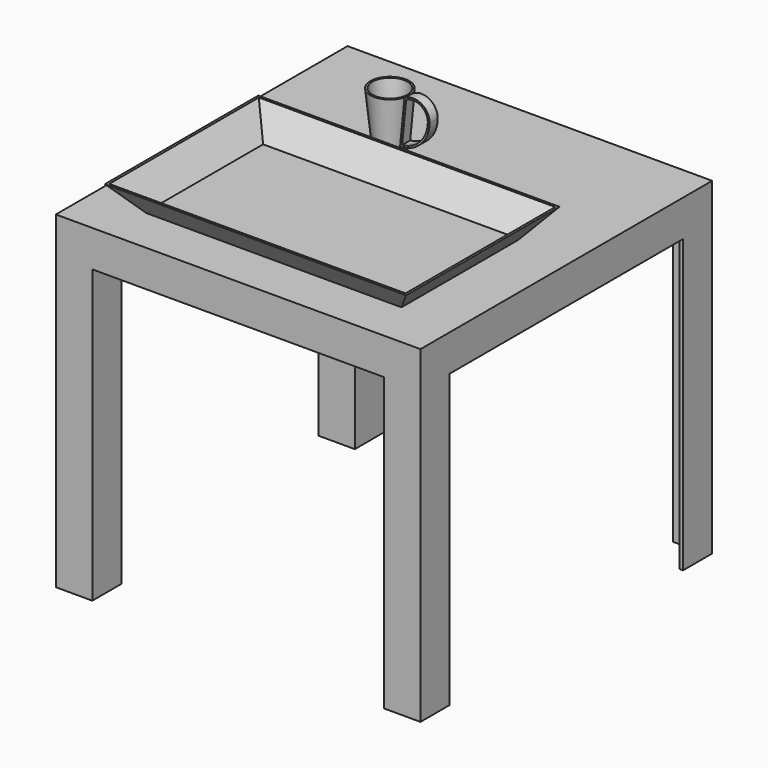
from build123d import *

# Parameters (mm, degrees)
F0_W         = 508
F0_H         = 457.2
F1_DEPTH     = 508
F3_DEPTH     = 406.4
F4_T         = 5.08
F4_T3_DEPTH  = 60.96
F4_T5_DEPTH  = 60.96
F4_T7_DEPTH  = 60.96
F4_T9_DEPTH  = 60.96
F5_R         = 19.05
F6_DEPTH     = 76.2
F6_TAPER     = -6
F7_T         = 2.54
F7_T3_DEPTH  = 55.88
F7_T5_DEPTH  = 55.88
F7_T7_DEPTH  = 55.88
F7_T9_DEPTH  = 10.16
F7_T11_DEPTH = 10.16
F7_T13_DEPTH = 55.88
F7_T15_DEPTH = 10.16
F7_T17_DEPTH = 457.2
F7_T19_DEPTH = 416.56
F7_T21_DEPTH = 411.48
F7_T23_DEPTH = 45.72
F7_T25_DEPTH = 452.12
F7_T27_DEPTH = 502.92
F7_T29_DEPTH = 502.92
F7_T31_DEPTH = 45.72
F7_T33_DEPTH = 416.56
F7_T35_DEPTH = 421.64
F7_T37_DEPTH = 421.64
F7_T39_DEPTH = 45.72
F7_T41_DEPTH = 45.72
F9_DEPTH     = 171.57005
F10_DEPTH    = 157.48264
F11_T        = -2.54
F12_W        = 355.6
F12_H        = 203.2
F13_DEPTH    = 38.1
F13_TAPER    = -40
F14_T        = -2.54


# Not quite as in the source:
# - a shell that OpenCascade refuses in one call is made with other operations: the cavity is built on its own and cut out


with BuildPart() as f1:
    # F0 (on Front) → F1 (new body)
    with BuildSketch(Plane.XZ):
        with Locations((2.3560058326, 45.4168599456)):
            Rectangle(F0_W, F0_H)
    extrude(amount=F1_DEPTH)

    # F2 (on face) → F3 (cut)
    with BuildSketch(Plane(origin=(0, 0, -183.1831400544), x_dir=(1, 0, 0), z_dir=(0, 0, -1))):
        Polygon((-200.8439941674, 457.2), (-251.6439941674, 457.2), (-251.6439941674, 50.8), (-200.8439941674, 50.8), (-200.8439941674, 0), (205.5560058326, 0), (205.5560058326, 50.8), (256.3560058326, 50.8), (256.3560058326, 457.2), (205.5560058326, 457.2), (205.5560058326, 508), (-200.8439941674, 508), align=None)
    extrude(amount=-F3_DEPTH, mode=Mode.SUBTRACT)

    # F4: shell of thickness 5.08, made by hand


with BuildPart() as f4_core1:
    # F4_t2: copy of F1
    add(f1.part)

    # the walls: a layer under each face that stays
    f4_faces = [f4_core1.faces().sort_by_distance(p)[0] for p in [
        (256.3560058326, -471.7142857143, -150.5259971973),
        (-215.3582798817, 0, -150.5259971973),
        (2.3560058326, -254, 274.0168599456),
        (-215.3582798817, -508, -150.5259971973),
        (230.9560058326, -482.6, -183.1831400544),
        (230.9560058326, -457.2, 20.0168599456),
        (2.3560058326, -254, 223.2168599456),
        (-200.8439941674, -25.4, 20.0168599456),
        (-226.2439941674, -25.4, -183.1831400544),
        (-251.6439941674, -471.7142857143, 241.3597170885),
        (205.5560058326, -482.6, 20.0168599456),
        (-200.8439941674, -482.6, 20.0168599456),
        (-226.2439941674, -482.6, -183.1831400544),
        (-226.2439941674, -457.2, 20.0168599456),
        (-226.2439941674, -50.8, 20.0168599456),
    ]]
    thicken(f4_faces, amount=-F4_T, mode=Mode.SUBTRACT)

    # F4_s4 → F4_t3 (cut)
    with BuildSketch(Plane.YZ.offset(200.4760058326)):
        Polygon((-457.1492, 223.1660599456), (-462.28, 223.2168599456), (-462.28, 228.2968599456), (-457.2, 228.2968599456), align=None)
    extrude(amount=F4_T3_DEPTH, mode=Mode.SUBTRACT)

    # F4_s6 → F4_t5 (cut)
    with BuildSketch(Plane.YZ.offset(-256.7239941674)):
        Polygon((-457.1492, 223.1660599456), (-457.2, 228.2968599456), (-462.28, 228.2968599456), (-462.28, 223.2168599456), align=None)
        Polygon((-50.8508, 223.1660599456), (-50.8, 228.2968599456), (-45.72, 228.2968599456), (-45.72, 223.2168599456), align=None)
    extrude(amount=F4_T5_DEPTH, mode=Mode.SUBTRACT)

    # F4_s8 → F4_t7 (cut)
    with BuildSketch(Plane.XZ.offset(-5.08)):
        Polygon((-200.7931941674, 223.1660599456), (-200.8439941674, 228.2968599456), (-205.9239941674, 228.2968599456), (-205.9239941674, 223.2168599456), align=None)
    extrude(amount=F4_T7_DEPTH, mode=Mode.SUBTRACT)

    # F4_s10 → F4_t9 (cut)
    with BuildSketch(Plane.XZ.offset(452.12)):
        Polygon((205.5052058326, 223.1660599456), (205.5560058326, 228.2968599456), (210.6360058326, 228.2968599456), (210.6360058326, 223.2168599456), align=None)
        Polygon((-200.7931941674, 223.1660599456), (-200.8439941674, 228.2968599456), (-205.9239941674, 228.2968599456), (-205.9239941674, 223.2168599456), align=None)
    extrude(amount=F4_T9_DEPTH, mode=Mode.SUBTRACT)


with BuildPart() as f1_1:
    add(f1.part)

    # what is left inside the walls is the cavity
    f4_cavity = [f4_core1.part.solids().sort_by_distance(p)[0] for p in [
        (2.356006, -336.973333, 268.88606),
    ]]
    add(f4_cavity, mode=Mode.SUBTRACT)

    # F5 (on face) → F6 (join)
    with BuildSketch(Plane.XY.offset(274.0168599456)):
        with Locations((-62.2486248612, -162.9570871592)):
            Circle(F5_R)
    extrude(amount=F6_DEPTH, taper=F6_TAPER)

    # F7: shell of thickness 2.54, made by hand


with BuildPart() as f7_core1:
    # F7_t2: copy of F1
    add(f1_1.part)

    # the walls: a layer under each face that stays
    f7_faces = [f7_core1.faces().sort_by_distance(p)[0] for p in [
        (256.3560058326, -471.7142857143, -150.5259971973),
        (-215.3582798817, 0, -150.5259971973),
        (2.3560058326, -254, 274.0168599456),
        (-215.3582798817, -508, -150.5259971973),
        (230.9560058326, -482.6, -183.1831400544),
        (230.9560058326, -457.2, 20.0168599456),
        (2.3560058326, -254, 223.2168599456),
        (253.8160058326, -50.8, 20.0168599456),
        (209.1845772611, -3.6285714286, -183.1831400544),
        (205.5560058326, -2.54, 20.0168599456),
        (-200.8439941674, -25.4, 20.0168599456),
        (-226.2439941674, -25.4, -183.1831400544),
        (-251.6439941674, -471.7142857143, 241.3597170885),
        (-85.3030962249, -162.9570871592, 312.1168599456),
        (205.5560058326, -482.6, 20.0168599456),
        (-200.8439941674, -482.6, 20.0168599456),
        (-226.2439941674, -482.6, -183.1831400544),
        (-226.2439941674, -457.2, 20.0168599456),
        (-226.2439941674, -50.8, 20.0168599456),
        (205.5560058326, -27.94, 225.7568599456),
        (228.4160058326, -50.8, 225.7568599456),
        (251.2760058326, -467.36, -150.8888543401),
        (-211.0039941674, -5.08, -150.8888543401),
        (2.3560058326, -254, 228.2968599456),
        (230.9560058326, -462.28, 25.0968599456),
        (230.9560058326, -482.6, -178.1031400544),
        (-211.0039941674, -502.92, -146.171711483),
        (2.3560058326, -254, 268.9368599456),
        (-246.5639941674, -467.36, 237.0054313742),
        (-226.2439941674, -25.4, -178.1031400544),
        (-205.9239941674, -25.4, 25.0968599456),
        (210.6360058326, -482.6, 25.0968599456),
        (-226.2439941674, -45.72, 25.0968599456),
        (-226.2439941674, -462.28, 25.0968599456),
        (-205.9239941674, -482.6, 25.0968599456),
        (-226.2439941674, -482.6, -178.1031400544),
    ]]
    thicken(f7_faces, amount=-F7_T, mode=Mode.SUBTRACT)

    # F7_s4 → F7_t3 (cut)
    with BuildSketch(Plane.YZ.offset(203.0160058326)):
        Polygon((-457.1746, 223.1914599456), (-459.74, 223.2168599456), (-459.74, 225.7568599456), (-457.2, 225.7568599456), align=None)
    extrude(amount=F7_T3_DEPTH, mode=Mode.SUBTRACT)

    # F7_s6 → F7_t5 (cut)
    with BuildSketch(Plane.YZ.offset(-254.1839941674)):
        Polygon((-457.1746, 223.1914599456), (-457.2, 225.7568599456), (-459.74, 225.7568599456), (-459.74, 223.2168599456), align=None)
        Polygon((-50.8254, 223.1914599456), (-50.8, 225.7568599456), (-48.26, 225.7568599456), (-48.26, 223.2168599456), align=None)
    extrude(amount=F7_T5_DEPTH, mode=Mode.SUBTRACT)

    # F7_s8 → F7_t7 (cut)
    with BuildSketch(Plane.XZ.offset(-2.54)):
        Polygon((-200.8185941674, 223.1914599456), (-200.8439941674, 225.7568599456), (-203.3839941674, 225.7568599456), (-203.3839941674, 223.2168599456), align=None)
    extrude(amount=F7_T7_DEPTH, mode=Mode.SUBTRACT)

    # F7_s10 → F7_t9 (cut)
    with BuildSketch(Plane.XZ.offset(-2.54)):
        Polygon((205.5306058326, 223.1914599456), (205.5560058326, 225.7568599456), (208.0960058326, 225.7568599456), (208.0960058326, 223.2168599456), align=None)
    extrude(amount=F7_T9_DEPTH, mode=Mode.SUBTRACT)

    # F7_s12 → F7_t11 (cut)
    with BuildSketch(Plane.YZ.offset(248.7360058326)):
        Polygon((-50.8254, 223.1914599456), (-50.8, 225.7568599456), (-48.26, 225.7568599456), (-48.26, 223.2168599456), align=None)
    extrude(amount=F7_T11_DEPTH, mode=Mode.SUBTRACT)

    # F7_s14 → F7_t13 (cut)
    with BuildSketch(Plane.XZ.offset(454.66)):
        Polygon((205.5306058326, 223.1914599456), (205.5560058326, 225.7568599456), (208.0960058326, 225.7568599456), (208.0960058326, 223.2168599456), align=None)
        Polygon((-200.8185941674, 223.1914599456), (-200.8439941674, 225.7568599456), (-203.3839941674, 225.7568599456), (-203.3839941674, 223.2168599456), align=None)
    extrude(amount=F7_T13_DEPTH, mode=Mode.SUBTRACT)

    # F7_s16 → F7_t15 (cut)
    with BuildSketch(Plane.XY.offset(220.6768599456)):
        Polygon((205.5814058326, -50.7746), (203.0160058326, -50.8), (203.0160058326, -53.34), (205.5560058326, -53.34), align=None)
        Polygon((205.5814058326, -5.1054), (203.0160058326, -5.08), (203.0160058326, -2.54), (205.5560058326, -2.54), align=None)
        Polygon((251.2506058326, -50.7746), (251.2760058326, -53.34), (253.8160058326, -53.34), (253.8160058326, -50.8), align=None)
    extrude(amount=F7_T15_DEPTH, mode=Mode.SUBTRACT)

    # F7_s18 → F7_t17 (cut)
    with BuildSketch(Plane.XY.offset(-185.7231400544)):
        Polygon((251.2506058326, -5.1054), (253.8160058326, -5.08), (253.8160058326, -2.54), (251.2760058326, -2.54), align=None)
    extrude(amount=F7_T17_DEPTH, mode=Mode.SUBTRACT)

    # F7_s20 → F7_t19 (cut)
    with BuildSketch(Plane.XZ.offset(48.26)):
        Polygon((251.2506058326, 228.3222599456), (253.8160058326, 228.2968599456), (253.8160058326, 225.7568599456), (251.2760058326, 225.7568599456), align=None)
    extrude(amount=F7_T19_DEPTH, mode=Mode.SUBTRACT)

    # F7_s22 → F7_t21 (cut)
    with BuildSketch(Plane.XY.offset(-180.6431400544)):
        Polygon((251.2506058326, -462.3054), (253.8160058326, -462.28), (253.8160058326, -459.74), (251.2760058326, -459.74), align=None)
        Polygon((-205.9493941674, -5.1054), (-205.9239941674, -2.54), (-203.3839941674, -2.54), (-203.3839941674, -5.08), align=None)
        Polygon((210.6614058326, -462.3054), (210.6360058326, -459.74), (208.0960058326, -459.74), (208.0960058326, -462.28), align=None)
        Polygon((210.6614058326, -502.8946), (210.6360058326, -505.46), (208.0960058326, -505.46), (208.0960058326, -502.92), align=None)
        Polygon((-205.9493941674, -502.8946), (-205.9239941674, -505.46), (-203.3839941674, -505.46), (-203.3839941674, -502.92), align=None)
        Polygon((-246.5385941674, -462.3054), (-249.1039941674, -462.28), (-249.1039941674, -459.74), (-246.5639941674, -459.74), align=None)
        Polygon((-246.5385941674, -45.6946), (-249.1039941674, -45.72), (-249.1039941674, -48.26), (-246.5639941674, -48.26), align=None)
        Polygon((-205.9493941674, -45.6946), (-203.3839941674, -45.72), (-203.3839941674, -48.26), (-205.9239941674, -48.26), align=None)
        Polygon((-205.9493941674, -462.3054), (-205.9239941674, -459.74), (-203.3839941674, -459.74), (-203.3839941674, -462.28), align=None)
    extrude(amount=F7_T21_DEPTH, mode=Mode.SUBTRACT)

    # F7_s24 → F7_t23 (cut)
    with BuildSketch(Plane.XZ.offset(459.74)):
        Polygon((251.2506058326, -178.0777400544), (253.8160058326, -178.1031400544), (253.8160058326, -180.6431400544), (251.2760058326, -180.6431400544), align=None)
        Polygon((210.6614058326, -178.0777400544), (210.6360058326, -180.6431400544), (208.0960058326, -180.6431400544), (208.0960058326, -178.1031400544), align=None)
        Polygon((-246.5385941674, -178.0777400544), (-249.1039941674, -178.1031400544), (-249.1039941674, -180.6431400544), (-246.5639941674, -180.6431400544), align=None)
        Polygon((-205.9493941674, -178.0777400544), (-203.3839941674, -178.1031400544), (-203.3839941674, -180.6431400544), (-205.9239941674, -180.6431400544), align=None)
    extrude(amount=F7_T23_DEPTH, mode=Mode.SUBTRACT)

    # F7_s26 → F7_t25 (cut)
    with BuildSketch(Plane.XY.offset(-180.6431400544)):
        Polygon((251.2506058326, -502.8946), (253.8160058326, -502.92), (253.8160058326, -505.46), (251.2760058326, -505.46), align=None)
        Polygon((-246.5385941674, -5.1054), (-246.5639941674, -2.54), (-249.1039941674, -2.54), (-249.1039941674, -5.08), align=None)
        Polygon((-246.5385941674, -502.8946), (-246.5639941674, -505.46), (-249.1039941674, -505.46), (-249.1039941674, -502.92), align=None)
    extrude(amount=F7_T25_DEPTH, mode=Mode.SUBTRACT)

    # F7_s28 → F7_t27 (cut)
    with BuildSketch(Plane.XZ.offset(2.54)):
        Polygon((251.2506058326, 268.9114599456), (253.8160058326, 268.9368599456), (253.8160058326, 271.4768599456), (251.2760058326, 271.4768599456), align=None)
        Polygon((-246.5385941674, 268.9114599456), (-246.5639941674, 271.4768599456), (-249.1039941674, 271.4768599456), (-249.1039941674, 268.9368599456), align=None)
    extrude(amount=F7_T27_DEPTH, mode=Mode.SUBTRACT)

    # F7_s30 → F7_t29 (cut)
    with BuildSketch(Plane.YZ.offset(-249.1039941674)):
        Polygon((-5.1054, 268.9114599456), (-2.54, 268.9368599456), (-2.54, 271.4768599456), (-5.08, 271.4768599456), align=None)
        Polygon((-502.8946, 268.9114599456), (-505.46, 268.9368599456), (-505.46, 271.4768599456), (-502.92, 271.4768599456), align=None)
    extrude(amount=F7_T29_DEPTH, mode=Mode.SUBTRACT)

    # F7_s32 → F7_t31 (cut)
    with BuildSketch(Plane.YZ.offset(-249.1039941674)):
        Polygon((-5.1054, -178.0777400544), (-2.54, -178.1031400544), (-2.54, -180.6431400544), (-5.08, -180.6431400544), align=None)
        Polygon((-502.8946, -178.0777400544), (-505.46, -178.1031400544), (-505.46, -180.6431400544), (-502.92, -180.6431400544), align=None)
        Polygon((-45.6946, -178.0777400544), (-45.72, -180.6431400544), (-48.26, -180.6431400544), (-48.26, -178.1031400544), align=None)
        Polygon((-462.3054, -178.0777400544), (-459.74, -178.1031400544), (-459.74, -180.6431400544), (-462.28, -180.6431400544), align=None)
    extrude(amount=F7_T31_DEPTH, mode=Mode.SUBTRACT)

    # F7_s34 → F7_t33 (cut)
    with BuildSketch(Plane.YZ.offset(-208.4639941674)):
        Polygon((-5.1054, 228.3222599456), (-2.54, 228.2968599456), (-2.54, 225.7568599456), (-5.08, 225.7568599456), align=None)
    extrude(amount=F7_T33_DEPTH, mode=Mode.SUBTRACT)

    # F7_s36 → F7_t35 (cut)
    with BuildSketch(Plane.YZ.offset(-208.4639941674)):
        Polygon((-502.8946, 228.3222599456), (-502.92, 225.7568599456), (-505.46, 225.7568599456), (-505.46, 228.2968599456), align=None)
    extrude(amount=F7_T35_DEPTH, mode=Mode.SUBTRACT)

    # F7_s38 → F7_t37 (cut)
    with BuildSketch(Plane.XZ.offset(43.18)):
        Polygon((-246.5385941674, 228.3222599456), (-246.5639941674, 225.7568599456), (-249.1039941674, 225.7568599456), (-249.1039941674, 228.2968599456), align=None)
    extrude(amount=F7_T37_DEPTH, mode=Mode.SUBTRACT)

    # F7_s40 → F7_t39 (cut)
    with BuildSketch(Plane.YZ.offset(208.0960058326)):
        Polygon((-462.3054, -178.0777400544), (-459.74, -178.1031400544), (-459.74, -180.6431400544), (-462.28, -180.6431400544), align=None)
        Polygon((-502.8946, -178.0777400544), (-502.92, -180.6431400544), (-505.46, -180.6431400544), (-505.46, -178.1031400544), align=None)
    extrude(amount=F7_T39_DEPTH, mode=Mode.SUBTRACT)

    # F7_s42 → F7_t41 (cut)
    with BuildSketch(Plane.XZ.offset(2.54)):
        Polygon((-246.5385941674, -178.0777400544), (-249.1039941674, -178.1031400544), (-249.1039941674, -180.6431400544), (-246.5639941674, -180.6431400544), align=None)
        Polygon((-205.9493941674, -178.0777400544), (-205.9239941674, -180.6431400544), (-203.3839941674, -180.6431400544), (-203.3839941674, -178.1031400544), align=None)
    extrude(amount=F7_T41_DEPTH, mode=Mode.SUBTRACT)

    # F7_s43 → F7_t44 (revolve, cut)
    with BuildSketch(Plane.XZ.offset(162.9570871592)):
        Polygon((-43.1733640051, 274.0396049226), (-43.1986248612, 271.4768599456), (-46.0195806489, 271.4768599456), (-45.7247104755, 274.2823622423), align=None)
    revolve(axis=Axis((-62.2486248612, -162.9570871592, 274.0168599456), (0, 0, 1)), mode=Mode.SUBTRACT)


with BuildPart() as f1_2:
    add(f1_1.part)

    # what is left inside the walls is the cavity
    f7_cavity = [f7_core1.part.solids().sort_by_distance(p)[0] for p in [
        (-81.407624, -162.957087, 299.596516),
    ]]
    add(f7_cavity, mode=Mode.SUBTRACT)


with BuildPart() as f9:
    # F8 (on Front) → F9 (new body)
    with BuildSketch(Plane.XZ):
        with BuildLine():
            Line((-35.106454912, 350.4484652221), (-41.1830060184, 289.0078127384))
            ThreePointArc((-41.1830060184, 289.0078127384), (-11.9988867349, 301.7594494347), (0, 331.2610387802))
            ThreePointArc((0, 331.2610387802), (-11.8635539237, 351.2649165915), (-35.106454912, 350.4484652221))
        make_face()
    extrude(amount=F9_DEPTH)

    # F8 (on Front) → F10 (cut)
    with BuildSketch(Plane.XZ):
        with BuildLine():
            Line((-35.106454912, 350.4484652221), (-41.1830060184, 289.0078127384))
            ThreePointArc((-41.1830060184, 289.0078127384), (-11.9988867349, 301.7594494347), (0, 331.2610387802))
            ThreePointArc((0, 331.2610387802), (-11.8635539237, 351.2649165915), (-35.106454912, 350.4484652221))
        make_face()
    extrude(amount=F10_DEPTH, mode=Mode.SUBTRACT)

    # F11
    f11_openings = [f9.faces().sort_by_distance(p)[0] for p in [
        (-21.605171, -157.48264, 323.102128),
        (-21.605171, -171.57005, 323.102128),
    ]]
    offset(amount=F11_T, openings=f11_openings)


with BuildPart() as f13:
    # F12 (on face) → F13 (new body)
    with BuildSketch(Plane.XY.offset(274.0168599456)):
        with Locations((0.8842647076, -342.3638771056)):
            Rectangle(F12_W, F12_H)
    extrude(amount=F13_DEPTH, taper=F13_TAPER)

    # F14
    f14_openings = [f13.faces().sort_by_distance(p)[0] for p in [
        (0.884265, -342.363877, 312.11686),
    ]]
    offset(amount=F14_T, openings=f14_openings, kind=Kind.INTERSECTION)


solid = Compound([f1_2.part, f9.part, f13.part])
